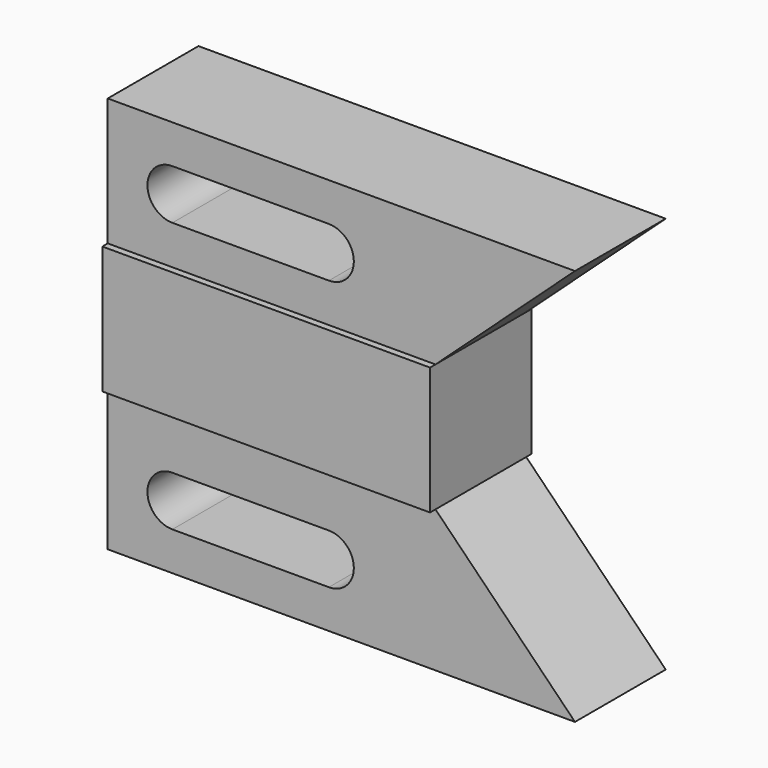
from build123d import *

# Parameters (mm, degrees)
F0_W     = 73.406
F0_H     = 28.575
F1_DEPTH = 25.4
F2_W     = 73.406
F2_H     = 28.575
F3_DEPTH = 1.524
F4_W     = 73.406
F4_H     = 28.575
F5_DEPTH = 1.524


with BuildPart() as f1:
    # F0 (on Front) → F1 (new body)
    with BuildSketch(Plane.XZ):
        Polygon((0, 31.75), (0, 0), (104.648, 0), (73.406, 31.75), align=None)
        with BuildLine():
            Line((49.53, 8.636), (14.478, 8.636))
            ThreePointArc((14.478, 8.636), (8.89, 14.224), (14.478, 19.812))
            Line((14.478, 19.812), (49.53, 19.812))
            ThreePointArc((49.53, 19.812), (55.118, 14.224), (49.53, 8.636))
        make_face(mode=Mode.SUBTRACT)
        with Locations((36.703, 46.0375)):
            Rectangle(F0_W, F0_H)
        Polygon((0, 88.9), (0, 60.325), (73.406, 60.325), (104.648, 88.9), align=None)
        with BuildLine():
            Line((49.53, 69.088), (14.478, 69.088))
            ThreePointArc((14.478, 69.088), (8.89, 74.676), (14.478, 80.264))
            Line((14.478, 80.264), (49.53, 80.264))
            ThreePointArc((49.53, 80.264), (55.118, 74.676), (49.53, 69.088))
        make_face(mode=Mode.SUBTRACT)
    extrude(amount=F1_DEPTH)

    # F2 (on face) → F3 (join)
    with BuildSketch(Plane.XZ.offset(25.4)):
        with Locations((36.703, 46.0375)):
            Rectangle(F2_W, F2_H)
    extrude(amount=F3_DEPTH)

    # F4 (on face) → F5 (join)
    with BuildSketch(Plane(origin=(0, 0, 0), x_dir=(-1, 0, 0), z_dir=(0, 1, 0))):
        with Locations((-36.703, 46.0375)):
            Rectangle(F4_W, F4_H)
    extrude(amount=F5_DEPTH)


solid = f1.part
